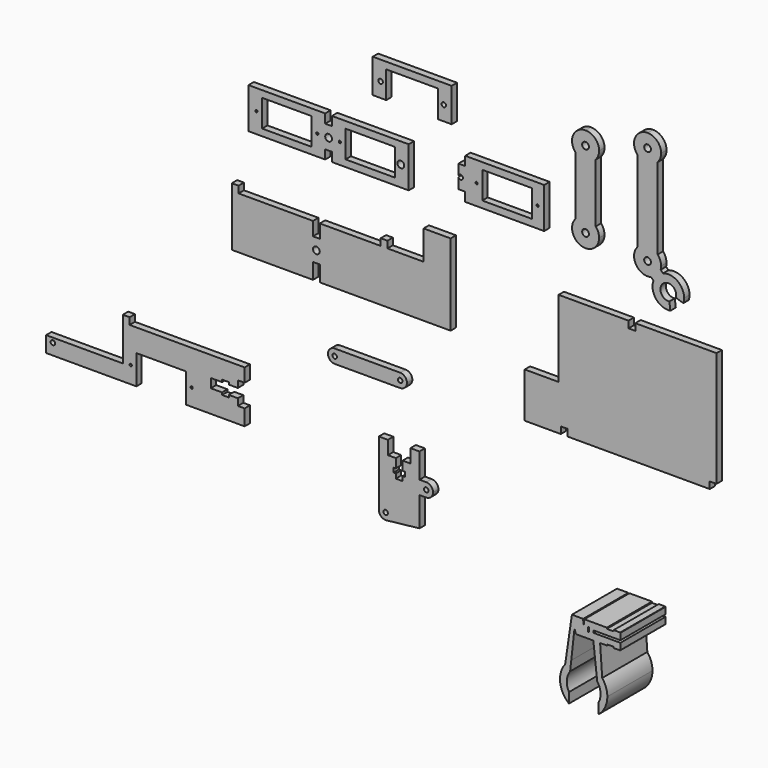
from build123d import *

# Parameters (mm, degrees)
F1_DEPTH  = 3
F3_DEPTH  = 3
F4_R      = 0.5
F4_W      = 22
F4_H      = 12
F4_R_2    = 1.5
F5_DEPTH  = 3
F7_DEPTH  = 3
F8_R      = 0.5
F9_DEPTH  = 25
F10_R     = 1
F11_DEPTH = 25
F13_DEPTH = 3
F14_R     = 1
F14_R_2   = 0.5
F15_DEPTH = 25
F17_DEPTH = 3
F18_R     = 1
F19_DEPTH = 3
F21_DEPTH = 3
F23_DEPTH = 3
F24_W     = 6
F24_H     = 3
F24_W_2   = 23
F25_DEPTH = 3
F26_W     = 0.5
F26_H     = 2
F27_DEPTH = 25


with BuildPart() as f1:
    # F0 (on Front) → F1 (new body)
    with BuildSketch(Plane.XZ):
        Polygon((31, 0), (0, 0), (0, -34), (-15, -34), (-15, -54), (1, -54), (1, -51), (4, -51), (4, -54), (67, -54), (67, -51), (70, -51), (70, 0), (34, 0), (34, -3), (31, -3), align=None)
    extrude(amount=F1_DEPTH)


with BuildPart() as f3:
    # F2 (on Front) → F3 (new body)
    with BuildSketch(Plane.XZ):
        Polygon((-105.8383033276, -29.5556988567), (-47.8383033276, -29.5556988567), (-47.8383033276, 6.4443011433), (-58.7832847834, 6.4443011433), (-59.8383033276, 6.4443011433), (-59.8383033276, 4.4443011433), (-59.8383033276, -6.5556988567), (-75.8383033276, -6.5556988567), (-75.8383033276, -3.5556988567), (-78.8383033276, -3.5556988567), (-78.8383033276, -6.5556988567), (-105.8383033276, -6.5556988567), (-105.8383033276, -12.5556988567), (-107.3383033276, -12.5556988567), (-108.8383033276, -12.5556988567), (-108.8383033276, -6.5556988567), (-141.8383033276, -6.5556988567), (-141.8383033276, -3.5556988567), (-144.8383033276, -3.5556988567), (-144.8383033276, -6.5556988567), (-144.8383033276, -29.5556988567), (-108.8383033276, -29.5556988567), (-108.8383033276, -22.5556988567), (-105.8383033276, -22.5556988567), align=None)
        with BuildLine():
            ThreePointArc((-105.8383033276, -17.5556988567), (-107.3383033276, -19.0556988567), (-108.8383033276, -17.5556988567))
            ThreePointArc((-108.8383033276, -17.5556988567), (-107.3383033276, -16.0556988567), (-105.8383033276, -17.5556988567))
        make_face(mode=Mode.SUBTRACT)
    extrude(amount=F3_DEPTH)


with BuildPart() as f5:
    # F4 (on Front) → F5 (new body)
    with BuildSketch(Plane.XZ):
        Polygon((-100.4267246723, 19.1396679729), (-66.4267246723, 19.1396679729), (-66.4267246723, 37.1396679729), (-69.9267246723, 37.1396679729), (-72.4267246723, 37.1396679729), (-100.4267246723, 37.1396679729), (-100.4267246723, 33.1396679729), (-103.4267246723, 33.1396679729), (-103.4267246723, 37.1396679729), (-131.4267246723, 37.1396679729), (-133.9267246723, 37.1396679729), (-137.4267246723, 37.1396679729), (-137.4267246723, 19.1396679729), (-103.4267246723, 19.1396679729), (-103.4267246723, 23.1396679729), (-100.4267246723, 23.1396679729), align=None)
        with Locations((-133.9267246723, 28.1396679729)):
            Circle(F4_R, mode=Mode.SUBTRACT)
        with Locations((-120.4267246723, 28.1396679729)):
            Rectangle(F4_W, F4_H, mode=Mode.SUBTRACT)
        with Locations((-106.9267246723, 28.1396679729)):
            Circle(F4_R, mode=Mode.SUBTRACT)
        with Locations((-101.9267246723, 28.1396679729)):
            Circle(F4_R_2, mode=Mode.SUBTRACT)
        with Locations((-96.9267246723, 28.1396679729)):
            Circle(F4_R, mode=Mode.SUBTRACT)
        with Locations((-83.4267246723, 28.1396679729)):
            Rectangle(F4_W, F4_H, mode=Mode.SUBTRACT)
        with Locations((-69.9267246723, 28.1396679729)):
            Circle(F4_R_2, mode=Mode.SUBTRACT)
    extrude(amount=F5_DEPTH)


with BuildPart() as f7:
    # F6 (on Front) → F7 (new body)
    with BuildSketch(Plane.XZ):
        Polygon((-11.8210216165, 31.7896194756), (-6.3822778761, 31.7896194756), (-6.3822778761, 40.7896194756), (-7.3822778761, 40.7896194756), (-9.3822778761, 40.7896194756), (-9.8822778761, 40.7896194756), (-12.3822778761, 40.7896194756), (-33.8210216165, 40.7896194756), (-36.3210216165, 40.7896194756), (-41.3822778761, 40.7896194756), (-41.3822778761, 36.7896194756), (-41.3822778761, 31.7896194756), (-34.9621884525, 31.7896194756), (-33.8210216165, 31.7896194756), (-33.8210216165, 37.7896194756), (-11.8210216165, 37.7896194756), align=None)
        Polygon((-41.3822778761, 22.7896194756), (-6.3822778761, 22.7896194756), (-6.3822778761, 31.7896194756), (-11.8210216165, 31.7896194756), (-11.8210216165, 25.7896194756), (-33.8210216165, 25.7896194756), (-33.8210216165, 31.7896194756), (-34.9621884525, 31.7896194756), (-41.3822778761, 31.7896194756), (-41.3822778761, 36.7896194756), (-44.3822778761, 36.7896194756), (-44.3822778761, 32.2521262616), (-44.3822778761, 26.7896194756), (-41.3822778761, 26.7896194756), align=None)
    extrude(amount=F7_DEPTH)

    # F8 (on face) → F9 (cut)
    with BuildSketch(Plane.XZ.offset(3)):
        with Locations((-36.3210216165, 31.7896194756)):
            Circle(F8_R)
        with Locations((-9.3210216165, 31.7896194756)):
            Circle(F8_R)
    extrude(amount=-F9_DEPTH, mode=Mode.SUBTRACT)

    # F10 (on face) → F11 (cut)
    with BuildSketch(Plane.XZ.offset(3)):
        with Locations((-43.4128455818, 31.7804962397)):
            Circle(F10_R)
    extrude(amount=-F11_DEPTH, mode=Mode.SUBTRACT)


with BuildPart() as f13:
    # F12 (on Front) → F13 (new body)
    with BuildSketch(Plane.XZ):
        Polygon((-227.1331846714, -89.5720042586), (-227.1331846714, -96.5720042586), (-187.1331846714, -96.5720042586), (-187.1331846714, -83.5720042586), (-165.1331846714, -83.5720042586), (-165.1331846714, -96.5720042586), (-139.1331846714, -96.5720042586), (-139.1331846714, -89.5720042586), (-142.1331846714, -89.5720042586), (-142.1331846714, -86.5720042586), (-146.1331846714, -86.5720042586), (-146.1331846714, -87.5720042586), (-149.1331846714, -87.5720042586), (-149.1331846714, -86.5720042586), (-154.1331846714, -86.5720042586), (-154.1331846714, -82.5720042586), (-149.1331846714, -82.5720042586), (-149.1331846714, -81.5720042586), (-146.1331846714, -81.5720042586), (-146.1331846714, -82.5720042586), (-142.1331846714, -82.5720042586), (-142.1331846714, -79.5720042586), (-139.1331846714, -79.5720042586), (-139.1331846714, -73.5720042586), (-190.1331846714, -73.5720042586), (-190.1331846714, -70.5720042586), (-193.1331846714, -70.5720042586), (-193.1331846714, -89.5720042586), align=None)
    extrude(amount=F13_DEPTH)

    # F14 (on face) → F15 (cut)
    with BuildSketch(Plane.XZ.offset(3)):
        with Locations((-224.1331846714, -91.5720042586)):
            Circle(F14_R)
        with Locations((-189.6331846714, -89.0720042586)):
            Circle(F14_R_2)
        with Locations((-162.6331846714, -89.0720042586)):
            Circle(F14_R_2)
    extrude(amount=-F15_DEPTH, mode=Mode.SUBTRACT)


with BuildPart() as f17:
    # F16 (on Front) → F17 (new body)
    with BuildSketch(Plane.XZ):
        with BuildLine():
            Line((-100.2078728676, -56.2117604315), (-102.2078728676, -56.2117604315))
            ThreePointArc((-102.2078728676, -56.2117604315), (-101.3291932111, -58.3330807751), (-99.2078728676, -59.2117604315))
            Line((-99.2078728676, -59.2117604315), (-70.2078728676, -59.2117604315))
            ThreePointArc((-70.2078728676, -59.2117604315), (-68.086552524, -58.3330807751), (-67.2078728676, -56.2117604315))
            Line((-67.2078728676, -56.2117604315), (-69.2078728676, -56.2117604315))
            ThreePointArc((-69.2078728676, -56.2117604315), (-70.2078728676, -57.2117604315), (-71.2078728676, -56.2117604315))
            Line((-71.2078728676, -56.2117604315), (-98.2078728676, -56.2117604315))
            ThreePointArc((-98.2078728676, -56.2117604315), (-99.2078728676, -57.2117604315), (-100.2078728676, -56.2117604315))
        make_face()
        with BuildLine():
            Line((-70.2078728676, -53.2117604315), (-99.2078728676, -53.2117604315))
            ThreePointArc((-99.2078728676, -53.2117604315), (-101.3291932111, -54.090440088), (-102.2078728676, -56.2117604315))
            Line((-102.2078728676, -56.2117604315), (-100.2078728676, -56.2117604315))
            ThreePointArc((-100.2078728676, -56.2117604315), (-99.2078728676, -55.2117604315), (-98.2078728676, -56.2117604315))
            Line((-98.2078728676, -56.2117604315), (-71.2078728676, -56.2117604315))
            ThreePointArc((-71.2078728676, -56.2117604315), (-70.2078728676, -55.2117604315), (-69.2078728676, -56.2117604315))
            Line((-69.2078728676, -56.2117604315), (-67.2078728676, -56.2117604315))
            ThreePointArc((-67.2078728676, -56.2117604315), (-68.086552524, -54.090440088), (-70.2078728676, -53.2117604315))
        make_face()
    extrude(amount=F17_DEPTH)


with BuildPart() as f19:
    # F18 (on Front) → F19 (new body)
    with BuildSketch(Plane.XZ):
        with BuildLine():
            Line((-72.1483585835, -87.1696201563), (-75.6483585835, -87.1696201563))
            Line((-75.6483585835, -87.1696201563), (-75.6483585835, -81.1696201563))
            Line((-75.6483585835, -81.1696201563), (-79.6483585835, -81.1696201563))
            Line((-79.6483585835, -81.1696201563), (-79.6483585835, -109.8178251102))
            ThreePointArc((-79.6483585835, -109.8178251102), (-78.6491229705, -112.0532091639), (-76.3170640052, -112.7994763143))
            Line((-76.3170640052, -112.7994763143), (-61.6483585835, -111.1696201563))
            Line((-61.6483585835, -111.1696201563), (-61.6483585835, -98.1696201563))
            Line((-61.6483585835, -98.1696201563), (-58.6483585835, -98.1696201563))
            ThreePointArc((-58.6483585835, -98.1696201563), (-56.5270382399, -97.2909404998), (-55.6483585835, -95.1696201563))
            ThreePointArc((-55.6483585835, -95.1696201563), (-56.5270382399, -93.0482998127), (-58.6483585835, -92.1696201563))
            Line((-58.6483585835, -92.1696201563), (-61.6483585835, -92.1696201563))
            Line((-61.6483585835, -92.1696201563), (-61.6483585835, -81.1696201563))
            Line((-61.6483585835, -81.1696201563), (-65.6483585835, -81.1696201563))
            Line((-65.6483585835, -81.1696201563), (-65.6483585835, -87.1696201563))
            Line((-65.6483585835, -87.1696201563), (-69.1483585835, -87.1696201563))
            Line((-69.1483585835, -87.1696201563), (-69.1483585835, -91.1696201563))
            Line((-69.1483585835, -91.1696201563), (-68.1483585835, -91.1696201563))
            Line((-68.1483585835, -91.1696201563), (-68.1483585835, -93.1696201563))
            Line((-68.1483585835, -93.1696201563), (-69.1483585835, -93.1696201563))
            Line((-69.1483585835, -93.1696201563), (-69.1483585835, -95.1696201563))
            Line((-69.1483585835, -95.1696201563), (-72.1483585835, -95.1696201563))
            Line((-72.1483585835, -95.1696201563), (-72.1483585835, -93.1696201563))
            Line((-72.1483585835, -93.1696201563), (-73.1483585835, -93.1696201563))
            Line((-73.1483585835, -93.1696201563), (-73.1483585835, -91.1696201563))
            Line((-73.1483585835, -91.1696201563), (-72.1483585835, -91.1696201563))
            Line((-72.1483585835, -91.1696201563), (-72.1483585835, -87.1696201563))
        make_face()
        with Locations((-76.6483585835, -109.8178251102)):
            Circle(F18_R, mode=Mode.SUBTRACT)
        with Locations((-58.6483585835, -95.1696201563)):
            Circle(F18_R, mode=Mode.SUBTRACT)
    extrude(amount=F19_DEPTH)


with BuildPart() as f21:
    # F20 (on Front) → F21 (new body)
    with BuildSketch(Plane.XZ):
        with BuildLine():
            Line((11.9623259716, 56.0655296445), (11.9623259716, 45.0655296445))
            Line((11.9623259716, 45.0655296445), (16.4623259716, 45.0655296445))
            Line((16.4623259716, 45.0655296445), (16.4623259716, 58.0969026779))
            ThreePointArc((16.4623259716, 58.0969026779), (14.4309529382, 56.5969026779), (11.9623259716, 56.0655296445))
        make_face()
        with BuildLine():
            Line((11.9623259716, 34.0655296445), (11.9623259716, 45.0655296445))
            Line((11.9623259716, 45.0655296445), (7.4623259716, 45.0655296445))
            Line((7.4623259716, 45.0655296445), (7.4623259716, 32.0341566111))
            ThreePointArc((7.4623259716, 32.0341566111), (9.493699005, 33.5341566111), (11.9623259716, 34.0655296445))
        make_face()
        with BuildLine():
            Line((16.4623259716, 45.0655296445), (11.9623259716, 45.0655296445))
            Line((11.9623259716, 45.0655296445), (11.9623259716, 34.0655296445))
            ThreePointArc((11.9623259716, 34.0655296445), (14.4309529382, 33.5341566111), (16.4623259716, 32.0341566111))
            Line((16.4623259716, 32.0341566111), (16.4623259716, 45.0655296445))
        make_face()
        with BuildLine():
            Line((7.4623259716, 45.0655296445), (11.9623259716, 45.0655296445))
            Line((11.9623259716, 45.0655296445), (11.9623259716, 56.0655296445))
            ThreePointArc((11.9623259716, 56.0655296445), (9.493699005, 56.5969026779), (7.4623259716, 58.0969026779))
            Line((7.4623259716, 58.0969026779), (7.4623259716, 45.0655296445))
        make_face()
        with BuildLine():
            ThreePointArc((16.4623259716, 32.0341566111), (14.4309529382, 33.5341566111), (11.9623259716, 34.0655296445))
            Line((11.9623259716, 34.0655296445), (11.9623259716, 29.5655296445))
            ThreePointArc((11.9623259716, 29.5655296445), (13.0229861434, 29.1261898163), (13.4623259716, 28.0655296445))
            ThreePointArc((13.4623259716, 28.0655296445), (13.0229861434, 27.0048694727), (11.9623259716, 26.5655296445))
            Line((11.9623259716, 26.5655296445), (11.9623259716, 22.0655296445))
            ThreePointArc((11.9623259716, 22.0655296445), (16.2049666587, 23.8228889574), (17.9623259716, 28.0655296445))
            ThreePointArc((17.9623259716, 28.0655296445), (17.5748120517, 30.186849988), (16.4623259716, 32.0341566111))
        make_face()
        with BuildLine():
            Line((11.9623259716, 29.5655296445), (11.9623259716, 34.0655296445))
            ThreePointArc((11.9623259716, 34.0655296445), (9.493699005, 33.5341566111), (7.4623259716, 32.0341566111))
            ThreePointArc((7.4623259716, 32.0341566111), (6.493699005, 25.5969026779), (11.9623259716, 22.0655296445))
            Line((11.9623259716, 22.0655296445), (11.9623259716, 26.5655296445))
            ThreePointArc((11.9623259716, 26.5655296445), (10.4623259716, 28.0655296445), (11.9623259716, 29.5655296445))
        make_face()
        with BuildLine():
            ThreePointArc((7.4623259716, 58.0969026779), (9.493699005, 56.5969026779), (11.9623259716, 56.0655296445))
            Line((11.9623259716, 56.0655296445), (11.9623259716, 60.5655296445))
            ThreePointArc((11.9623259716, 60.5655296445), (10.4623259716, 62.0655296445), (11.9623259716, 63.5655296445))
            Line((11.9623259716, 63.5655296445), (11.9623259716, 68.0655296445))
            ThreePointArc((11.9623259716, 68.0655296445), (6.493699005, 64.5341566111), (7.4623259716, 58.0969026779))
        make_face()
        with BuildLine():
            Line((11.9623259716, 60.5655296445), (11.9623259716, 56.0655296445))
            ThreePointArc((11.9623259716, 56.0655296445), (14.4309529382, 56.5969026779), (16.4623259716, 58.0969026779))
            ThreePointArc((16.4623259716, 58.0969026779), (17.5748120517, 59.9442093009), (17.9623259716, 62.0655296445))
            ThreePointArc((17.9623259716, 62.0655296445), (16.2049666587, 66.3081703316), (11.9623259716, 68.0655296445))
            Line((11.9623259716, 68.0655296445), (11.9623259716, 63.5655296445))
            ThreePointArc((11.9623259716, 63.5655296445), (13.0229861434, 63.1261898163), (13.4623259716, 62.0655296445))
            ThreePointArc((13.4623259716, 62.0655296445), (13.0229861434, 61.0048694727), (11.9623259716, 60.5655296445))
        make_face()
    extrude(amount=F21_DEPTH)


with BuildPart() as f23:
    # F22 (on Front) → F23 (new body)
    with BuildSketch(Plane.XZ):
        with BuildLine():
            Line((34.9792193533, 66.0388317555), (34.9513553083, 66.0388317555))
            Line((34.9513553083, 66.0388317555), (34.9513553083, 48.0388317555))
            Line((34.9513553083, 48.0388317555), (34.9513553083, 30.0388317555))
            Line((34.9513553083, 30.0388317555), (34.9792193533, 30.0388317555))
            ThreePointArc((34.9792193533, 30.0388317555), (39.4513553083, 32.0388317555), (43.9234912633, 30.0388317555))
            Line((43.9234912633, 30.0388317555), (43.9513553083, 30.0388317555))
            Line((43.9513553083, 30.0388317555), (43.9513553083, 48.0388317555))
            Line((43.9513553083, 48.0388317555), (43.9513553083, 66.0388317555))
            Line((43.9513553083, 66.0388317555), (43.9234912633, 66.0388317555))
            ThreePointArc((43.9234912633, 66.0388317555), (39.4513553083, 64.0388317555), (34.9792193533, 66.0388317555))
        make_face()
        with BuildLine():
            Line((43.9234912633, 66.0388317555), (34.9792193533, 66.0388317555))
            ThreePointArc((34.9792193533, 66.0388317555), (39.4513553083, 64.0388317555), (43.9234912633, 66.0388317555))
        make_face()
        with BuildLine():
            ThreePointArc((39.4513553083, 76.0388317555), (33.9741297332, 72.4883214983), (34.9792193533, 66.0388317555))
            Line((34.9792193533, 66.0388317555), (43.9234912633, 66.0388317555))
            ThreePointArc((43.9234912633, 66.0388317555), (45.0563894621, 67.8978992169), (45.4513553083, 70.0388317555))
            ThreePointArc((45.4513553083, 70.0388317555), (43.6939959954, 74.2814724426), (39.4513553083, 76.0388317555))
        make_face()
        with BuildLine():
            ThreePointArc((40.9513553083, 70.0388317555), (38.3906951365, 68.9781715837), (39.4513553083, 71.5388317555))
            ThreePointArc((39.4513553083, 71.5388317555), (40.5120154801, 71.0994919273), (40.9513553083, 70.0388317555))
        make_face(mode=Mode.SUBTRACT)
        with BuildLine():
            Line((43.9234912633, 30.0388317555), (34.9792193533, 30.0388317555))
            ThreePointArc((34.9792193533, 30.0388317555), (33.9741297332, 23.5893420127), (39.4513553083, 20.0388317555))
            Line((39.4513553083, 20.0388317555), (39.4513553083, 24.5388317555))
            ThreePointArc((39.4513553083, 24.5388317555), (38.3906951365, 27.0994919273), (40.9513553083, 26.0388317555))
            Line((40.9513553083, 26.0388317555), (45.4513553083, 26.0388317555))
            ThreePointArc((45.4513553083, 26.0388317555), (45.0563894621, 28.1797642942), (43.9234912633, 30.0388317555))
        make_face()
        with BuildLine():
            ThreePointArc((43.9234912633, 30.0388317555), (39.4513553083, 32.0388317555), (34.9792193533, 30.0388317555))
            Line((34.9792193533, 30.0388317555), (43.9234912633, 30.0388317555))
        make_face()
        with BuildLine():
            Line((39.4513553083, 24.5388317555), (39.4513553083, 20.0388317555))
            ThreePointArc((39.4513553083, 20.0388317555), (40.2345124616, 20.0901625873), (41.0042695789, 20.2432767978))
            ThreePointArc((41.0042695789, 20.2432767978), (42.4513553083, 20.8426793328), (43.6939959954, 21.7961910684))
            Line((43.6939959954, 21.7961910684), (40.5120154801, 24.9781715837))
            ThreePointArc((40.5120154801, 24.9781715837), (40.0253804568, 24.6530124568), (39.4513553083, 24.5388317555))
        make_face()
        with BuildLine():
            ThreePointArc((45.246910266, 24.4859174849), (45.4000244765, 25.2556746022), (45.4513553083, 26.0388317555))
            Line((45.4513553083, 26.0388317555), (40.9513553083, 26.0388317555))
            ThreePointArc((40.9513553083, 26.0388317555), (40.8371746071, 25.464806607), (40.5120154801, 24.9781715837))
            Line((40.5120154801, 24.9781715837), (43.6939959954, 21.7961910684))
            ThreePointArc((43.6939959954, 21.7961910684), (44.647507731, 23.0388317555), (45.246910266, 24.4859174849))
        make_face()
        with BuildLine():
            ThreePointArc((43.6939959954, 21.7961910684), (42.4513553083, 20.8426793328), (41.0042695789, 20.2432767978))
            Line((41.0042695789, 20.2432767978), (42.0502871652, 19.1972592115))
            ThreePointArc((42.0502871652, 19.1972592115), (42.7276636806, 20.5881009869), (43.6939959954, 21.7961910684))
        make_face()
        with BuildLine():
            Line((46.2929278523, 23.4398998987), (45.246910266, 24.4859174849))
            ThreePointArc((45.246910266, 24.4859174849), (44.647507731, 23.0388317555), (43.6939959954, 21.7961910684))
            ThreePointArc((43.6939959954, 21.7961910684), (44.9020860769, 22.7625233832), (46.2929278523, 23.4398998987))
        make_face()
        with BuildLine():
            ThreePointArc((46.2929278523, 23.4398998987), (44.9020860769, 22.7625233832), (43.6939959954, 21.7961910684))
            Line((43.6939959954, 21.7961910684), (44.5398034848, 20.950383579))
            Line((44.5398034848, 20.950383579), (46.6611238284, 23.0717039225))
            Line((46.6611238284, 23.0717039225), (46.2929278523, 23.4398998987))
        make_face()
        with BuildLine():
            Line((44.5398034848, 20.950383579), (43.6939959954, 21.7961910684))
            ThreePointArc((43.6939959954, 21.7961910684), (42.7276636806, 20.5881009869), (42.0502871652, 19.1972592115))
            Line((42.0502871652, 19.1972592115), (42.4184831413, 18.8290632354))
            Line((42.4184831413, 18.8290632354), (44.5398034848, 20.950383579))
        make_face()
        with BuildLine():
            Line((42.4184831413, 18.8290632354), (42.0502871652, 19.1972592115))
            ThreePointArc((42.0502871652, 19.1972592115), (43.2026685748, 12.4425017234), (49.5690134789, 9.9078648264))
            Line((49.5690134789, 9.9078648264), (49.1063784713, 13.3771542132))
            ThreePointArc((49.1063784713, 13.3771542132), (45.5059823231, 15.2958130753), (46.1688697296, 19.3213173342))
            Line((46.1688697296, 19.3213173342), (45.4513553083, 20.0388317555))
            Line((45.4513553083, 20.0388317555), (45.1082095578, 20.381977506))
            Line((45.1082095578, 20.381977506), (44.5398034848, 20.950383579))
            Line((44.5398034848, 20.950383579), (42.4184831413, 18.8290632354))
        make_face()
        with BuildLine():
            ThreePointArc((55.6437434637, 16.8464436001), (52.6776181965, 22.5672699949), (46.2929278523, 23.4398998987))
            Line((46.2929278523, 23.4398998987), (46.6611238284, 23.0717039225))
            Line((46.6611238284, 23.0717039225), (44.5398034848, 20.950383579))
            Line((44.5398034848, 20.950383579), (45.1082095578, 20.381977506))
            Line((45.1082095578, 20.381977506), (45.4513553083, 20.0388317555))
            Line((45.4513553083, 20.0388317555), (46.1688697296, 19.3213173342))
            ThreePointArc((46.1688697296, 19.3213173342), (49.983135477, 20.0800219639), (52.1437434637, 16.8464436001))
            ThreePointArc((52.1437434637, 16.8464436001), (52.102311646, 16.3095021429), (51.9789971046, 15.7852729488))
            Line((51.9789971046, 15.7852729488), (55.3142507454, 14.7241022975))
            ThreePointArc((55.3142507454, 14.7241022975), (55.5608798283, 15.7725606856), (55.6437434637, 16.8464436001))
        make_face()
    extrude(amount=F23_DEPTH)


with BuildPart() as f25:
    # F24 (on Front) → F25 (new body)
    with BuildSketch(Plane.XZ):
        Polygon((-80.3731644452, 56.1289462447), (-82.3731644452, 56.1289462447), (-82.3731644452, 51.1289462447), (-76.3731644452, 51.1289462447), (-76.3731644452, 56.1289462447), (-77.3731644452, 56.1289462447), (-78.8731644452, 56.1289462447), align=None)
        with BuildLine():
            Line((-76.3731644452, 56.1289462447), (-76.3731644452, 57.6289462447))
            Line((-76.3731644452, 57.6289462447), (-77.8731644452, 57.6289462447))
            ThreePointArc((-77.8731644452, 57.6289462447), (-78.166057664, 56.9218394635), (-78.8731644452, 56.6289462447))
            Line((-78.8731644452, 56.6289462447), (-78.8731644452, 56.1289462447))
            Line((-78.8731644452, 56.1289462447), (-77.3731644452, 56.1289462447))
            Line((-77.3731644452, 56.1289462447), (-76.3731644452, 56.1289462447))
        make_face()
        with BuildLine():
            Line((-76.3731644452, 63.1289462447), (-82.3731644452, 63.1289462447))
            Line((-82.3731644452, 63.1289462447), (-82.3731644452, 59.1289462447))
            Line((-82.3731644452, 59.1289462447), (-82.3731644452, 56.1289462447))
            Line((-82.3731644452, 56.1289462447), (-80.3731644452, 56.1289462447))
            Line((-80.3731644452, 56.1289462447), (-78.8731644452, 56.1289462447))
            Line((-78.8731644452, 56.1289462447), (-78.8731644452, 56.6289462447))
            ThreePointArc((-78.8731644452, 56.6289462447), (-79.5802712263, 58.3360530259), (-77.8731644452, 57.6289462447))
            Line((-77.8731644452, 57.6289462447), (-76.3731644452, 57.6289462447))
            Line((-76.3731644452, 57.6289462447), (-76.3731644452, 63.1289462447))
        make_face()
        with Locations((-79.3731644452, 64.6289462447)):
            Rectangle(F24_W, F24_H)
        with Locations((-64.8731644452, 64.6289462447)):
            Rectangle(F24_W_2, F24_H)
        with Locations((-50.3731644452, 64.6289462447)):
            Rectangle(F24_W, F24_H)
        with BuildLine():
            Line((-47.3731644452, 63.1289462447), (-53.3731644452, 63.1289462447))
            Line((-53.3731644452, 63.1289462447), (-53.3731644452, 57.6289462447))
            Line((-53.3731644452, 57.6289462447), (-51.8731644452, 57.6289462447))
            ThreePointArc((-51.8731644452, 57.6289462447), (-50.8731644452, 58.6289462447), (-49.8731644452, 57.6289462447))
            Line((-49.8731644452, 57.6289462447), (-47.3731644452, 57.6289462447))
            Line((-47.3731644452, 57.6289462447), (-47.3731644452, 63.1289462447))
        make_face()
        with BuildLine():
            Line((-47.3731644452, 56.1289462447), (-47.3731644452, 57.6289462447))
            Line((-47.3731644452, 57.6289462447), (-49.8731644452, 57.6289462447))
            ThreePointArc((-49.8731644452, 57.6289462447), (-50.166057664, 56.9218394635), (-50.8731644452, 56.6289462447))
            Line((-50.8731644452, 56.6289462447), (-50.8731644452, 56.1289462447))
            Line((-50.8731644452, 56.1289462447), (-47.3731644452, 56.1289462447))
        make_face()
        with BuildLine():
            Line((-51.8731644452, 57.6289462447), (-53.3731644452, 57.6289462447))
            Line((-53.3731644452, 57.6289462447), (-53.3731644452, 56.1289462447))
            Line((-53.3731644452, 56.1289462447), (-50.8731644452, 56.1289462447))
            Line((-50.8731644452, 56.1289462447), (-50.8731644452, 56.6289462447))
            ThreePointArc((-50.8731644452, 56.6289462447), (-51.5802712263, 56.9218394635), (-51.8731644452, 57.6289462447))
        make_face()
        Polygon((-50.8731644452, 56.1289462447), (-53.3731644452, 56.1289462447), (-53.3731644452, 51.1289462447), (-47.3731644452, 51.1289462447), (-47.3731644452, 56.1289462447), align=None)
    extrude(amount=F25_DEPTH)


with BuildPart() as f27:
    # F26 (on Front) → F27 (new body)
    with BuildSketch(Plane.XZ):
        with BuildLine():
            Line((32.2311602812, -108.2063924779), (33.0103132519, -115.2064226368))
            Line((33.0103132519, -115.2064226368), (36.0103132519, -115.2064226368))
            Line((36.0103132519, -115.2064226368), (39.0103238133, -115.2063924779))
            Line((39.0103238133, -115.2063924779), (39.0103238133, -114.7063924779))
            Line((39.0103238133, -114.7063924779), (42.0103238133, -114.7063924779))
            Line((42.0103238133, -114.7063924779), (42.0103238133, -115.2063924779))
            Line((42.0103238133, -115.2063924779), (44.8285043249, -115.2063924779))
            ThreePointArc((44.8285043249, -115.2063924779), (44.9570701181, -115.1531387827), (45.0103238133, -115.0245729895))
            Line((45.0103238133, -115.0245729895), (45.0103238133, -112.2063924779))
            Line((45.0103238133, -112.2063924779), (33.0103238133, -112.2063924779))
            Line((33.0103238133, -112.2063924779), (33.0103238133, -111.2063924779))
            Line((33.0103238133, -111.2063924779), (45.0103238133, -111.2063924779))
            Line((45.0103238133, -111.2063924779), (45.0103238133, -108.3882119663))
            ThreePointArc((45.0103238133, -108.3882119663), (44.9570701181, -108.2596461731), (44.8285043249, -108.2063924779))
            Line((44.8285043249, -108.2063924779), (42.0103238133, -108.2063924779))
            Line((42.0103238133, -108.2063924779), (42.0103238133, -108.7063924779))
            Line((42.0103238133, -108.7063924779), (39.0103238133, -108.7063924779))
            Line((39.0103238133, -108.7063924779), (39.0103238133, -108.2063924779))
            Line((39.0103238133, -108.2063924779), (36.0103238133, -108.2063924779))
            Line((36.0103238133, -108.2063924779), (32.2311602812, -108.2063924779))
        make_face()
        Polygon((25.2967402339, -115.2064226368), (33.0103132519, -115.2064226368), (32.2311602812, -108.2063924779), (29.0103238133, -108.2063924779), (28.6359283186, -111.5700192012), (28.5147354007, -108.2063924779), (25.2136614938, -108.2063924779), (24.655756368, -113.2186979599), align=None)
        with Locations((30.9199985415, -111.6092150807)):
            Rectangle(F26_W, F26_H, mode=Mode.SUBTRACT)
        with BuildLine():
            ThreePointArc((20.5295011666, -128.513191676), (21.7714482196, -127.2104248672), (23.217645376, -126.1389083597))
            Line((23.217645376, -126.1389083597), (24.434508523, -115.2064226368))
            Line((24.434508523, -115.2064226368), (24.655756368, -113.2186979599))
            Line((24.655756368, -113.2186979599), (25.2136614938, -108.2063924779))
            Line((25.2136614938, -108.2063924779), (23.5147354007, -108.2063924779))
            Line((23.5147354007, -108.2063924779), (20.5295011666, -128.513191676))
        make_face()
        with BuildLine():
            Line((33.0103132519, -115.2064226368), (34.227176399, -126.1389083597))
            ThreePointArc((34.227176399, -126.1389083597), (35.6889351318, -127.2241969495), (36.9412501367, -128.5456722785))
            Line((36.9412501367, -128.5456722785), (36.0103132519, -115.2064226368))
            Line((36.0103132519, -115.2064226368), (33.0103132519, -115.2064226368))
        make_face()
        with BuildLine():
            ThreePointArc((34.7213753455, -130.5788677256), (35.8372627283, -132.7077213457), (36.2224108875, -135.0802481174))
            ThreePointArc((36.2224108875, -135.0802481174), (35.9680992606, -137.0167397906), (35.2224108875, -138.8219055042))
            Line((35.2224108875, -138.8219055042), (35.2224108875, -143.3264593687))
            ThreePointArc((35.2224108875, -143.3264593687), (38.1696327013, -139.6628238124), (39.2224108875, -135.0802481174))
            ThreePointArc((39.2224108875, -135.0802481174), (38.6357305161, -131.6195987649), (36.9412501367, -128.5456722785))
            ThreePointArc((36.9412501367, -128.5456722785), (35.6889351318, -127.2241969495), (34.227176399, -126.1389083597))
            Line((34.227176399, -126.1389083597), (34.7213753455, -130.5788677256))
        make_face()
        with BuildLine():
            ThreePointArc((22.2224108875, -138.8219055042), (21.2362272078, -134.6252163442), (22.7234464295, -130.5788677256))
            Line((22.7234464295, -130.5788677256), (23.217645376, -126.1389083597))
            ThreePointArc((23.217645376, -126.1389083597), (21.7714482196, -127.2104248672), (20.5295011666, -128.513191676))
            ThreePointArc((20.5295011666, -128.513191676), (18.2903150314, -136.272462884), (22.2224108875, -143.3264593687))
            Line((22.2224108875, -143.3264593687), (22.2224108875, -138.8219055042))
        make_face()
    extrude(amount=F27_DEPTH)


solid = Compound([f1.part, f3.part, f5.part, f7.part, f13.part, f17.part, f19.part, f21.part, f23.part, f25.part, f27.part])
